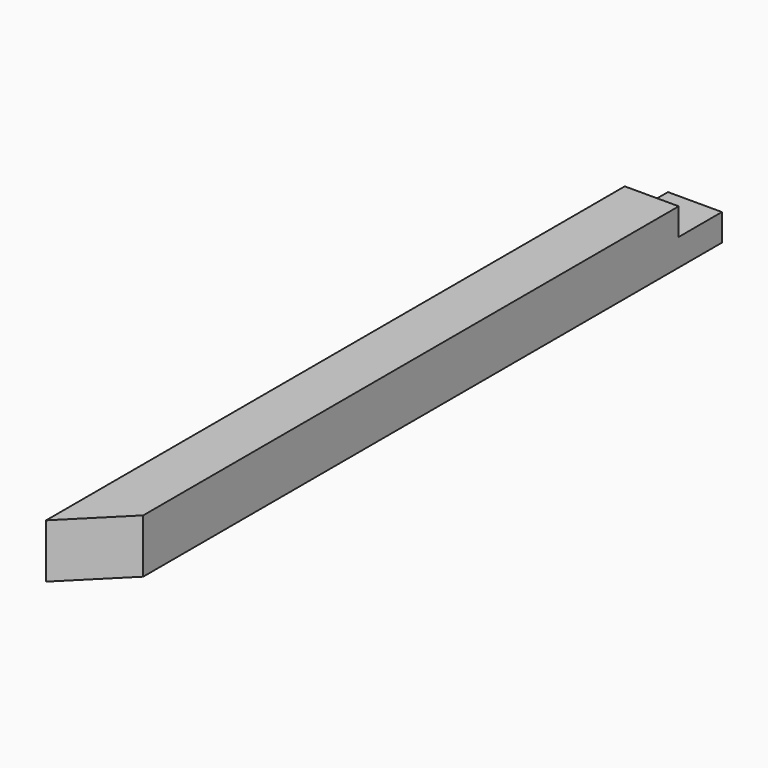
from build123d import *

# Parameters (mm, degrees)
F0_W     = 10
F0_H     = 10
F1_DEPTH = 144
F2_W     = 10
F2_H     = 5
F3_DEPTH = 10
F4_SIZE  = 9.99999


# Not quite as in the source:
# - a fillet or chamfer is up to 0.001 mm smaller than in the source, because OpenCascade refuses the exact size


with BuildPart() as f1:
    # F0 (on Front) → F1 (new body)
    with BuildSketch(Plane.XZ):
        Rectangle(F0_W, F0_H)
    extrude(amount=F1_DEPTH)

    # F2 (on face) → F3 (cut)
    with BuildSketch(Plane.YZ.offset(5)):
        with Locations((-5, 2.5)):
            Rectangle(F2_W, F2_H)
    extrude(amount=-F3_DEPTH, mode=Mode.SUBTRACT)

    # F4 (size 10 in the source; OpenCascade refuses exactly that, so slightly less here)
    f4_edges = [f1.edges().sort_by_distance(p)[0] for p in [
        (5, -144, 0),
    ]]
    chamfer(f4_edges, length=F4_SIZE)


solid = f1.part
